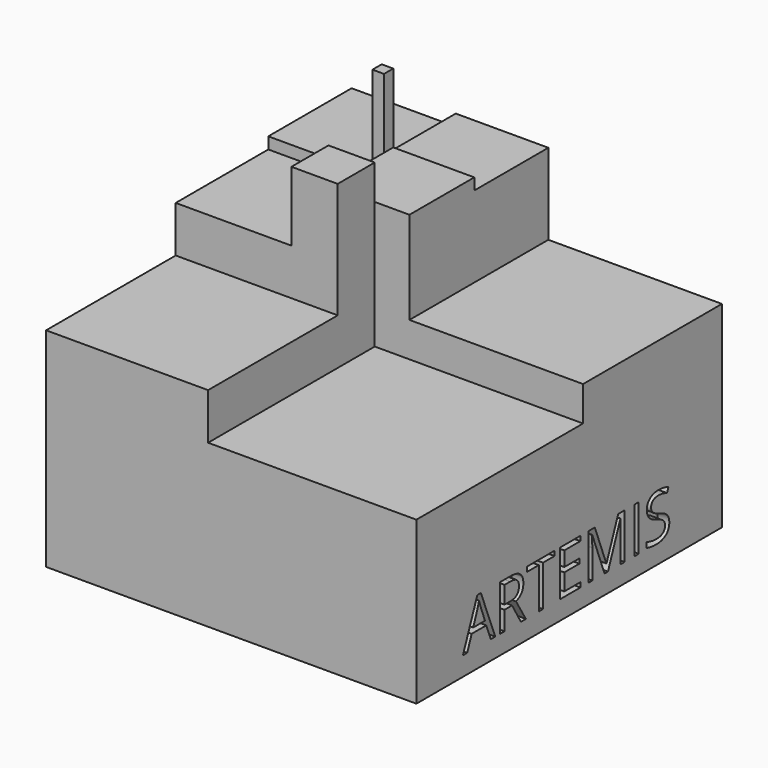
from build123d import *

# Parameters (mm, degrees)
F0_W          = 25.4
F0_H          = 25.4
F1_DEPTH      = 787.4
F2_DEPTH      = 584.2
F3_DEPTH      = 609.6
F4_DEPTH      = 431.8
F5_DEPTH      = 635
F6_DEPTH      = 558.8
F0_W_2        = 101.6
F0_H_2        = 101.6
F7_DEPTH      = 711.2
F8_DEPTH      = 457.2
F9_DEPTH      = 355.6
F10_TEXT_SIZE = 124.3143290695
F11_DEPTH     = 25.4
F12_TEXT_SIZE = 155.3900332914
F13_DEPTH     = 25.4
F14_TEXT_SIZE = 140.062543667
F15_DEPTH     = 25.4


# Not quite as in the source:
# - Text() gives the source's letters only with a copy of the font that has no kerning and outlines rounded to 1/6400 em; it was checked with that copy


with BuildPart() as f1:
    # F0 (on Top) → F1 (new body)
    with BuildSketch(Plane.XY):
        with Locations((-190.5, 97.0050433636)):
            Rectangle(F0_W, F0_H)
    extrude(amount=F1_DEPTH)

    # F0 (on Top) → F2 (join)
    with BuildSketch(Plane.XY):
        Polygon((-431.8, 84.3050433636), (-203.2, 84.3050433636), (-203.2, 109.7050433636), (-203.2, 312.9050433636), (-431.8, 312.9050433636), align=None)
    extrude(amount=F2_DEPTH)

    # F0 (on Top) → F3 (join)
    with BuildSketch(Plane.XY):
        Polygon((-177.8, 109.7050433636), (0, 109.7050433636), (0, 312.9050433636), (-203.2, 312.9050433636), (-203.2, 109.7050433636), align=None)
    extrude(amount=F3_DEPTH)

    # F0 (on Top) → F4 (join)
    with BuildSketch(Plane.XY):
        Polygon((0, 109.7050433636), (0, -68.0949566364), (381, -68.0949566364), (381, 312.9050433636), (0, 312.9050433636), align=None)
    extrude(amount=F4_DEPTH)

    # F0 (on Top) → F5 (join)
    with BuildSketch(Plane.XY):
        Polygon((-177.8, -68.0949566364), (-76.2, -68.0949566364), (0, -68.0949566364), (0, 109.7050433636), (-177.8, 109.7050433636), (-177.8, 84.3050433636), align=None)
    extrude(amount=F5_DEPTH)

    # F0 (on Top) → F6 (join)
    with BuildSketch(Plane.XY):
        Polygon((-177.8, -169.6949566364), (-177.8, -68.0949566364), (-177.8, 84.3050433636), (-203.2, 84.3050433636), (-431.8, 84.3050433636), (-431.8, -169.6949566364), align=None)
    extrude(amount=F6_DEPTH)

    # F0 (on Top) → F7 (join)
    with BuildSketch(Plane.XY):
        with Locations((-127, -118.8949566364)):
            Rectangle(F0_W_2, F0_H_2)
    extrude(amount=F7_DEPTH)

    # F0 (on Top) → F8 (join)
    with BuildSketch(Plane.XY):
        Polygon((-76.2, -525.2949566364), (-76.2, -169.6949566364), (-177.8, -169.6949566364), (-431.8, -169.6949566364), (-431.8, -525.2949566364), align=None)
    extrude(amount=F8_DEPTH)

    # F0 (on Top) → F9 (join)
    with BuildSketch(Plane.XY):
        Polygon((0, -68.0949566364), (-76.2, -68.0949566364), (-76.2, -169.6949566364), (-76.2, -525.2949566364), (381, -525.2949566364), (381, -68.0949566364), align=None)
    extrude(amount=F9_DEPTH)

    # F10 (on face) → F11 (cut)
    with BuildSketch(Plane(origin=(0, 312.9050433636, 0), x_dir=(-1, 0, 0), z_dir=(0, 1, 0))):
        with Locations((-293.3226525784, 40.2910225093)):
            Text('GSSE 2017', F10_TEXT_SIZE, font='Open Sans', text_align=(TextAlign.LEFT, TextAlign.BOTTOM))
    extrude(amount=-F11_DEPTH, mode=Mode.SUBTRACT)

    # F12 (on face) → F13 (cut)
    with BuildSketch(Plane(origin=(-431.8, 0, 0), x_dir=(0, -1, 0), z_dir=(-1, 0, 0))):
        with Locations((-131.990455091, 34.8636060953)):
            Text('ORION', F12_TEXT_SIZE, font='Open Sans', text_align=(TextAlign.LEFT, TextAlign.BOTTOM))
    extrude(amount=-F13_DEPTH, mode=Mode.SUBTRACT)

    # F14 (on face) → F15 (cut)
    with BuildSketch(Plane.YZ.offset(381)):
        with Locations((-397.695183754, 41.6328236461)):
            Text('ARTEMIS', F14_TEXT_SIZE, font='Open Sans', text_align=(TextAlign.LEFT, TextAlign.BOTTOM))
    extrude(amount=-F15_DEPTH, mode=Mode.SUBTRACT)


solid = f1.part
